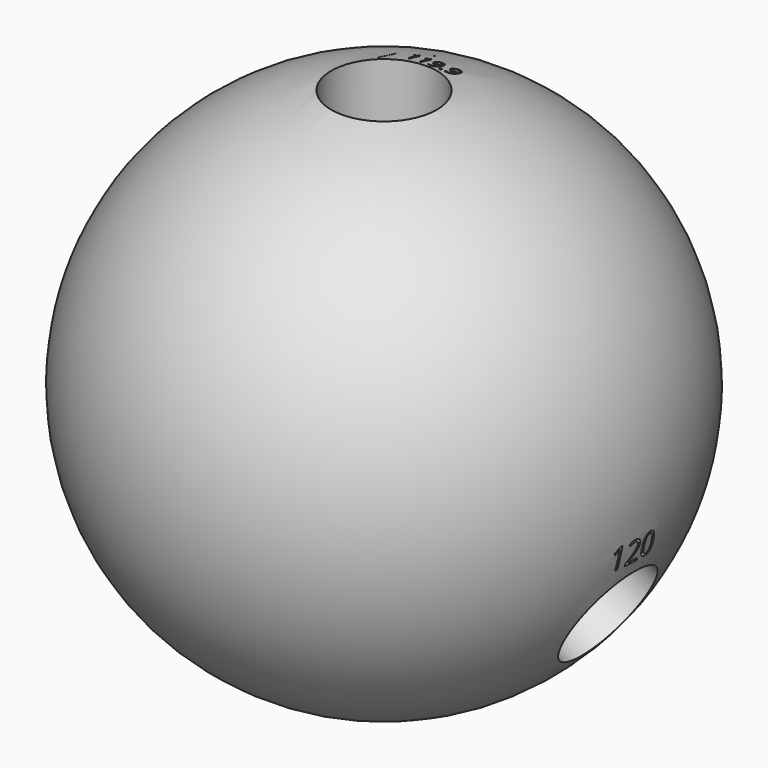
from build123d import *

# Parameters (mm, degrees)
F4_R          = 3.175
F5_DEPTH      = 25.4
F7_TEXT_SIZE  = 1.2162296722
F8_DEPTH      = 10.16
F10_ANGLE     = 120
F12_TEXT_SIZE = 2.5510545432
F13_DEPTH     = 10.16
F15_ANGLE     = -120
F17_TEXT_SIZE = 1.8669803265
F18_DEPTH     = 10.16


# Not quite as in the source:
# - Text() gives the source's letters only with a copy of the font that has no kerning and outlines rounded to 1/6400 em; it was checked with that copy


with BuildPart() as f2:
    # F0 (on Front) → F2 (revolve)
    with BuildSketch(Plane.XZ):
        with BuildLine():
            Line((15.875, 0), (-15.875, 0))
            ThreePointArc((-15.875, 0), (0, -15.875), (15.875, 0))
        make_face()
    revolve(axis=Axis((0, 0, 0), (1, 0, 0)))

    # F7 (on offset) → F8 (cut)
    with BuildSketch(Plane.XY.offset(19.05)):
        with Locations((-1.6284405137, 3.410235513)):
            Text('119.9', F7_TEXT_SIZE, font='Open Sans', text_align=(TextAlign.LEFT, TextAlign.BOTTOM))
    extrude(amount=-F8_DEPTH, mode=Mode.SUBTRACT)

    # F12 (on offset) → F13 (cut)
    with BuildSketch(Plane(origin=(-16.4977839421, 0, -9.525), x_dir=(0, -1, 0), z_dir=(-0.8660254038, 0, -0.5))):
        with Locations((-2.2282695863, 3.6903510336)):
            Text('120', F12_TEXT_SIZE, font='Open Sans', text_align=(TextAlign.LEFT, TextAlign.BOTTOM))
    extrude(amount=-F13_DEPTH, mode=Mode.SUBTRACT)

    # F17 (on offset) → F18 (cut)
    with BuildSketch(Plane(origin=(16.4977839421, 0, -9.525), x_dir=(0, 1, 0), z_dir=(0.8660254038, 0, -0.5))):
        with Locations((-2.1310982411, 3.8957800716)):
            Text('120', F17_TEXT_SIZE, font='Open Sans', text_align=(TextAlign.LEFT, TextAlign.BOTTOM))
    extrude(amount=-F18_DEPTH, mode=Mode.SUBTRACT)


with BuildPart() as f5:
    # F4 (on offset) → F5 (new body)
    with BuildSketch(Plane.XY.offset(6.35)):
        Circle(F4_R)
    extrude(amount=F5_DEPTH)


with BuildPart() as f10_1:
    # F10: copy of F5
    add(f5.part.rotate(Axis((0, -4.8854034394, 0), (0, -1, 0)), F10_ANGLE))


with BuildPart() as f15_1:
    # F15: copy of F5
    add(f5.part.rotate(Axis((0, 14.5640317351, 0), (0, -1, 0)), F15_ANGLE))


with BuildPart() as f2_1:
    add(f2.part)

    # F19: cut F5, F15_1, F10_1
    add(f5.part, mode=Mode.SUBTRACT)
    add(f15_1.part, mode=Mode.SUBTRACT)
    add(f10_1.part, mode=Mode.SUBTRACT)


solid = f2_1.part
